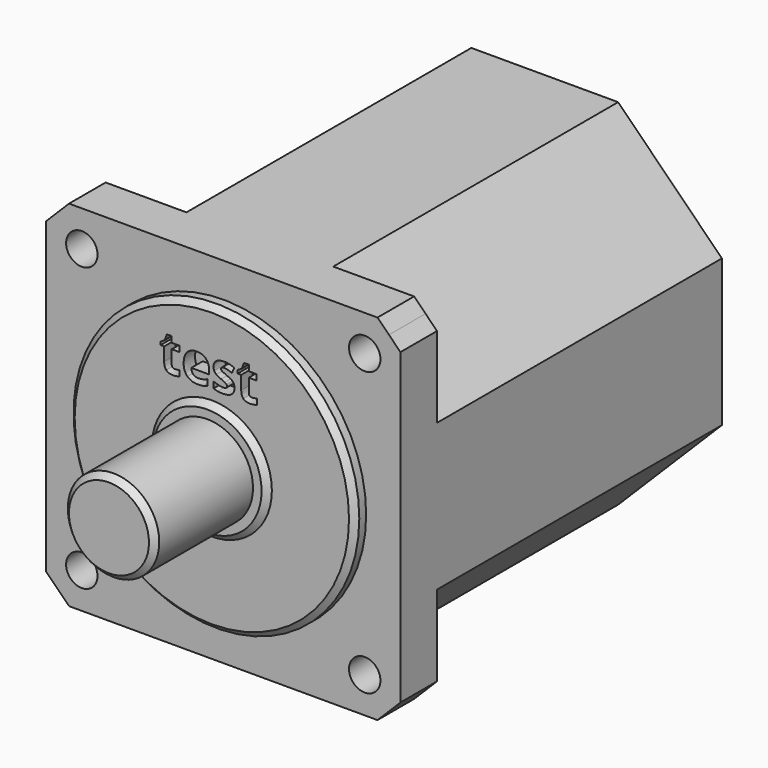
from build123d import *

# Parameters (mm, degrees)
F1_DEPTH  = 70.3
F2_DEPTH  = 62.3
F3_DEPTH  = 62.3
F4_R      = 2.75
F5_DEPTH  = 8
F4_R_2    = 25
F4_R_3    = 8
F6_DEPTH  = 2.5
F7_DEPTH  = 70.301
F8_R      = 10.5
F8_R_2    = 8
F9_DEPTH  = 1
F10_SIZE  = 0.99999
F11_SIZE  = 1
F12_DEPTH = 25
F13_SIZE  = 1


# Not quite as in the source:
# - a fillet or chamfer is up to 0.001 mm smaller than in the source, because OpenCascade refuses the exact size


with BuildPart() as f1:
    # F0 (on Front) → F1 (new body)
    with BuildSketch(Plane.XZ):
        Polygon((12.841, -31), (31, -31), (31, -12.841), align=None)
        Polygon((-12.841, -31), (12.841, -31), (31, -12.841), (31, 12.841), (12.841, 31), (-12.841, 31), (-31, 12.841), (-31, -12.841), align=None)
        Polygon((-31, -31), (-12.841, -31), (-31, -12.841), align=None)
        Polygon((12.841, 31), (31, 12.841), (31, 31), align=None)
        Polygon((-31, 31), (-31, 12.841), (-12.841, 31), align=None)
    extrude(amount=F1_DEPTH)

    # F0 (on Front) → F2 (cut)
    with BuildSketch(Plane.XZ):
        Polygon((12.841, 31), (31, 12.841), (31, 31), align=None)
    extrude(amount=F2_DEPTH, mode=Mode.SUBTRACT)

    # F0 (on Front) → F3 (cut)
    with BuildSketch(Plane.XZ):
        Polygon((-31, 31), (-31, 12.841), (-12.841, 31), align=None)
        Polygon((-31, -31), (-12.841, -31), (-31, -12.841), align=None)
        Polygon((12.841, -31), (31, -31), (31, -12.841), align=None)
    extrude(amount=F3_DEPTH, mode=Mode.SUBTRACT)

    # F4 (on face) → F5 (cut)
    with BuildSketch(Plane.XZ.offset(70.3)):
        with Locations((-24.7487373415, 24.7487373415)):
            Circle(F4_R)
        with Locations((24.7487373415, 24.7487373415)):
            Circle(F4_R)
        with Locations((24.7487373415, -24.7487373415)):
            Circle(F4_R)
        with Locations((-24.7487373415, -24.7487373415)):
            Circle(F4_R)
    extrude(amount=-F5_DEPTH, mode=Mode.SUBTRACT)

    # F4 (on face) → F6 (join)
    with BuildSketch(Plane.XZ.offset(70.3)):
        Circle(F4_R_2)
        with BuildLine():
            add(Edge.make_bspline(
                [(-6.8632484674, 13.3325467897), (-6.7054646432, 13.1982921323), (-6.4452597403, 13.1982921323)],
                knots=[0, 0, 0, 1, 1, 1], degree=2))
            add(Edge.make_bspline(
                [(-6.4452597403, 13.1982921323), (-6.099242582, 13.1982921323), (-5.6148185605, 13.3491556133)],
                knots=[0, 0, 0, 1, 1, 1], degree=2))
            Line((-5.6148185605, 13.3491556133), (-5.6148185605, 12.3678509525))
            add(Edge.make_bspline(
                [(-5.6148185605, 12.3678509525), (-6.1075469938, 12.1463999712), (-6.8258786143, 12.1463999712)],
                knots=[0, 0, 0, 1, 1, 1], degree=2))
            add(Edge.make_bspline(
                [(-6.8258786143, 12.1463999712), (-7.6175658724, 12.1463999712), (-7.9788077855, 12.5470878405)],
                knots=[0, 0, 0, 1, 1, 1], degree=2))
            add(Edge.make_bspline(
                [(-7.9788077855, 12.5470878405), (-8.3400496987, 12.9477757097), (-8.3400496987, 13.7477673796)],
                knots=[0, 0, 0, 1, 1, 1], degree=2))
            Line((-8.3400496987, 13.7477673796), (-8.3400496987, 16.0785389574))
            Line((-8.3400496987, 16.0785389574), (-8.9711849954, 16.0785389574))
            Line((-8.9711849954, 16.0785389574), (-8.9711849954, 16.6363186165))
            Line((-8.9711849954, 16.6363186165), (-8.2445489631, 17.0778365104))
            Line((-8.2445489631, 17.0778365104), (-7.863930089, 18.0992791615))
            Line((-7.863930089, 18.0992791615), (-7.0210322916, 18.0992791615))
            Line((-7.0210322916, 18.0992791615), (-7.0210322916, 17.0695320986))
            Line((-7.0210322916, 17.0695320986), (-5.6674131685, 17.0695320986))
            Line((-5.6674131685, 17.0695320986), (-5.6674131685, 16.0785389574))
            Line((-5.6674131685, 16.0785389574), (-7.0210322916, 16.0785389574))
            Line((-7.0210322916, 16.0785389574), (-7.0210322916, 13.7477673796))
            add(Edge.make_bspline(
                [(-7.0210322916, 13.7477673796), (-7.0210322916, 13.4668014471), (-6.8632484674, 13.3325467897)],
                knots=[0, 0, 0, 1, 1, 1], degree=2))
        make_face(mode=Mode.SUBTRACT)
        with BuildLine():
            add(Edge.make_bspline(
                [(-1.4889099657, 12.2308281579), (-1.8819854575, 12.1463999712), (-2.449453597, 12.1463999712)],
                knots=[0, 0, 0, 1, 1, 1], degree=2))
            add(Edge.make_bspline(
                [(-2.449453597, 12.1463999712), (-3.6162234545, 12.1463999712), (-4.2736560552, 12.7913759542)],
                knots=[0, 0, 0, 1, 1, 1], degree=2))
            add(Edge.make_bspline(
                [(-4.2736560552, 12.7913759542), (-4.9310886558, 13.4363519371), (-4.9310886558, 14.616962481)],
                knots=[0, 0, 0, 1, 1, 1], degree=2))
            add(Edge.make_bspline(
                [(-4.9310886558, 14.616962481), (-4.9310886558, 15.8321747408), (-4.323482526, 16.4958356503)],
                knots=[0, 0, 0, 1, 1, 1], degree=2))
            add(Edge.make_bspline(
                [(-4.323482526, 16.4958356503), (-3.7158763961, 17.1594965597), (-2.6432232056, 17.1594965597)],
                knots=[0, 0, 0, 1, 1, 1], degree=2))
            add(Edge.make_bspline(
                [(-2.6432232056, 17.1594965597), (-1.6190124172, 17.1594965597), (-1.0480841061, 16.576111631)],
                knots=[0, 0, 0, 1, 1, 1], degree=2))
            add(Edge.make_bspline(
                [(-1.0480841061, 16.576111631), (-0.477155795, 15.9927267022), (-0.477155795, 14.9629796393)],
                knots=[0, 0, 0, 1, 1, 1], degree=2))
            Line((-0.477155795, 14.9629796393), (-0.477155795, 14.3221558622))
            Line((-0.477155795, 14.3221558622), (-3.595462425, 14.3221558622))
            add(Edge.make_bspline(
                [(-3.595462425, 14.3221558622), (-3.5733173269, 13.7602239972), (-3.2619018845, 13.4446563489)],
                knots=[0, 0, 0, 1, 1, 1], degree=2))
            add(Edge.make_bspline(
                [(-3.2619018845, 13.4446563489), (-2.9504864421, 13.1290887006), (-2.3885545771, 13.1290887006)],
                knots=[0, 0, 0, 1, 1, 1], degree=2))
            add(Edge.make_bspline(
                [(-2.3885545771, 13.1290887006), (-1.9511888891, 13.1290887006), (-1.5622656032, 13.2197451961)],
                knots=[0, 0, 0, 1, 1, 1], degree=2))
            add(Edge.make_bspline(
                [(-1.5622656032, 13.2197451961), (-1.1733423174, 13.3104016915), (-0.7498173157, 13.5097075747)],
                knots=[0, 0, 0, 1, 1, 1], degree=2))
            Line((-0.7498173157, 13.5097075747), (-0.7498173157, 12.4882649236))
            add(Edge.make_bspline(
                [(-0.7498173157, 12.4882649236), (-1.0958344739, 12.3152563445), (-1.4889099657, 12.2308281579)],
                knots=[0, 0, 0, 1, 1, 1], degree=2))
        make_face(mode=Mode.SUBTRACT)
        Circle(F4_R_3, mode=Mode.SUBTRACT)
        with BuildLine():
            add(Edge.make_bspline(
                [(3.843906477, 14.2882461807), (3.9698567226, 14.028733312), (3.9698567226, 13.6702595361)],
                knots=[0, 0, 0, 1, 1, 1], degree=2))
            add(Edge.make_bspline(
                [(3.9698567226, 13.6702595361), (3.9698567226, 12.9256306116), (3.4529070882, 12.5360152914)],
                knots=[0, 0, 0, 1, 1, 1], degree=2))
            add(Edge.make_bspline(
                [(3.4529070882, 12.5360152914), (2.9359574538, 12.1463999712), (1.9062103909, 12.1463999712)],
                knots=[0, 0, 0, 1, 1, 1], degree=2))
            add(Edge.make_bspline(
                [(1.9062103909, 12.1463999712), (1.3788802417, 12.1463999712), (1.0065657795, 12.2183715402)],
                knots=[0, 0, 0, 1, 1, 1], degree=2))
            add(Edge.make_bspline(
                [(1.0065657795, 12.2183715402), (0.6342513172, 12.2903431091), (0.3103792571, 12.4287499724)],
                knots=[0, 0, 0, 1, 1, 1], degree=2))
            Line((0.3103792571, 12.4287499724), (0.3103792571, 13.5180119865))
            add(Edge.make_bspline(
                [(0.3103792571, 13.5180119865), (0.6771574448, 13.3450034074), (1.1380522996, 13.2280496079)],
                knots=[0, 0, 0, 1, 1, 1], degree=2))
            add(Edge.make_bspline(
                [(1.1380522996, 13.2280496079), (1.5989471544, 13.1110958084), (1.9491165185, 13.1110958084)],
                knots=[0, 0, 0, 1, 1, 1], degree=2))
            add(Edge.make_bspline(
                [(1.9491165185, 13.1110958084), (2.667448139, 13.1110958084), (2.667448139, 13.5263163983)],
                knots=[0, 0, 0, 1, 1, 1], degree=2))
            add(Edge.make_bspline(
                [(2.667448139, 13.5263163983), (2.667448139, 13.6827161538), (2.5719474033, 13.7802929924)],
                knots=[0, 0, 0, 1, 1, 1], degree=2))
            add(Edge.make_bspline(
                [(2.5719474033, 13.7802929924), (2.4764466677, 13.877869831), (2.243231103, 14.0010519394)],
                knots=[0, 0, 0, 1, 1, 1], degree=2))
            add(Edge.make_bspline(
                [(2.243231103, 14.0010519394), (2.0100155384, 14.1242340477), (1.6210922525, 14.2875541464)],
                knots=[0, 0, 0, 1, 1, 1], degree=2))
            add(Edge.make_bspline(
                [(1.6210922525, 14.2875541464), (1.0633125934, 14.5214617454), (0.8010315875, 14.7207676285)],
                knots=[0, 0, 0, 1, 1, 1], degree=2))
            add(Edge.make_bspline(
                [(0.8010315875, 14.7207676285), (0.5387505816, 14.9200735117), (0.4204127134, 15.1775102774)],
                knots=[0, 0, 0, 1, 1, 1], degree=2))
            add(Edge.make_bspline(
                [(0.4204127134, 15.1775102774), (0.3020748453, 15.4349470431), (0.3020748453, 15.8100296426)],
                knots=[0, 0, 0, 1, 1, 1], degree=2))
            add(Edge.make_bspline(
                [(0.3020748453, 15.8100296426), (0.3020748453, 16.4550056256), (0.8010315875, 16.8072510927)],
                knots=[0, 0, 0, 1, 1, 1], degree=2))
            add(Edge.make_bspline(
                [(0.8010315875, 16.8072510927), (1.2999883297, 17.1594965597), (2.2176258333, 17.1594965597)],
                knots=[0, 0, 0, 1, 1, 1], degree=2))
            add(Edge.make_bspline(
                [(2.2176258333, 17.1594965597), (3.0909731407, 17.1594965597), (3.9172621146, 16.7788776857)],
                knots=[0, 0, 0, 1, 1, 1], degree=2))
            Line((3.9172621146, 16.7788776857), (3.5200344169, 15.8280225349))
            add(Edge.make_bspline(
                [(3.5200344169, 15.8280225349), (3.1560243664, 15.9830382217), (2.8404567181, 16.0826911633)],
                knots=[0, 0, 0, 1, 1, 1], degree=2))
            add(Edge.make_bspline(
                [(2.8404567181, 16.0826911633), (2.5248890698, 16.1823441049), (2.1954807352, 16.1823441049)],
                knots=[0, 0, 0, 1, 1, 1], degree=2))
            add(Edge.make_bspline(
                [(2.1954807352, 16.1823441049), (1.6114037721, 16.1823441049), (1.6114037721, 15.8667764566)],
                knots=[0, 0, 0, 1, 1, 1], degree=2))
            add(Edge.make_bspline(
                [(1.6114037721, 15.8667764566), (1.6114037721, 15.6896156716), (1.7996371062, 15.5595132201)],
                knots=[0, 0, 0, 1, 1, 1], degree=2))
            add(Edge.make_bspline(
                [(1.7996371062, 15.5595132201), (1.9878704402, 15.4294107686), (2.6245420114, 15.1747421401)],
                knots=[0, 0, 0, 1, 1, 1], degree=2))
            add(Edge.make_bspline(
                [(2.6245420114, 15.1747421401), (3.1906260823, 14.944986747), (3.4542911568, 14.7463728982)],
                knots=[0, 0, 0, 1, 1, 1], degree=2))
            add(Edge.make_bspline(
                [(3.4542911568, 14.7463728982), (3.7179562314, 14.5477590494), (3.843906477, 14.2882461807)],
                knots=[0, 0, 0, 1, 1, 1], degree=2))
        make_face(mode=Mode.SUBTRACT)
        with BuildLine():
            add(Edge.make_bspline(
                [(6.6175800174, 13.3325467897), (6.7753638416, 13.1982921323), (7.0355687446, 13.1982921323)],
                knots=[0, 0, 0, 1, 1, 1], degree=2))
            add(Edge.make_bspline(
                [(7.0355687446, 13.1982921323), (7.3815859028, 13.1982921323), (7.8660099243, 13.3491556133)],
                knots=[0, 0, 0, 1, 1, 1], degree=2))
            Line((7.8660099243, 13.3491556133), (7.8660099243, 12.3678509525))
            add(Edge.make_bspline(
                [(7.8660099243, 12.3678509525), (7.373281491, 12.1463999712), (6.6549498705, 12.1463999712)],
                knots=[0, 0, 0, 1, 1, 1], degree=2))
            add(Edge.make_bspline(
                [(6.6549498705, 12.1463999712), (5.8632626125, 12.1463999712), (5.5020206993, 12.5470878405)],
                knots=[0, 0, 0, 1, 1, 1], degree=2))
            add(Edge.make_bspline(
                [(5.5020206993, 12.5470878405), (5.1407787861, 12.9477757097), (5.1407787861, 13.7477673796)],
                knots=[0, 0, 0, 1, 1, 1], degree=2))
            Line((5.1407787861, 13.7477673796), (5.1407787861, 16.0785389574))
            Line((5.1407787861, 16.0785389574), (4.5096434895, 16.0785389574))
            Line((4.5096434895, 16.0785389574), (4.5096434895, 16.6363186165))
            Line((4.5096434895, 16.6363186165), (5.2362795217, 17.0778365104))
            Line((5.2362795217, 17.0778365104), (5.6168983958, 18.0992791615))
            Line((5.6168983958, 18.0992791615), (6.4597961933, 18.0992791615))
            Line((6.4597961933, 18.0992791615), (6.4597961933, 17.0695320986))
            Line((6.4597961933, 17.0695320986), (7.8134153163, 17.0695320986))
            Line((7.8134153163, 17.0695320986), (7.8134153163, 16.0785389574))
            Line((7.8134153163, 16.0785389574), (6.4597961933, 16.0785389574))
            Line((6.4597961933, 16.0785389574), (6.4597961933, 13.7477673796))
            add(Edge.make_bspline(
                [(6.4597961933, 13.7477673796), (6.4597961933, 13.4668014471), (6.6175800174, 13.3325467897)],
                knots=[0, 0, 0, 1, 1, 1], degree=2))
        make_face(mode=Mode.SUBTRACT)
    extrude(amount=F6_DEPTH)

    # F4 (on face) → F7 (cut, through all)
    with BuildSketch(Plane.XZ.offset(70.3)):
        Polygon((26.9827560573, 31), (28.9913780286, 28.9913780286), (31, 26.9827560573), (31, 31), align=None)
        Polygon((31, -31), (31, -26.9827560573), (28.9913780286, -28.9913780286), (26.9827560573, -31), align=None)
        Polygon((-31, -31), (-26.9827560573, -31), (-28.9913780286, -28.9913780286), (-31, -26.9827560573), align=None)
        Polygon((-28.9913780286, 28.9913780286), (-26.9827560573, 31), (-31, 31), (-31, 26.9827560573), align=None)
    extrude(amount=-F7_DEPTH, mode=Mode.SUBTRACT)

    # F8 (on face) → F9 (join)
    with BuildSketch(Plane.XZ.offset(72.8)):
        Circle(F8_R)
        Circle(F8_R_2, mode=Mode.SUBTRACT)
    extrude(amount=F9_DEPTH)

    # F10 (size 1 in the source; OpenCascade refuses exactly that, so slightly less here)
    f10_edges = [f1.edges().sort_by_distance(p)[0] for p in [
        (-10.5, -73.8, 0),
    ]]
    chamfer(f10_edges, length=F10_SIZE)

    # F11
    f11_edges = [f1.edges().sort_by_distance(p)[0] for p in [
        (-25, -72.8, 0),
    ]]
    chamfer(f11_edges, length=F11_SIZE)

    # F4 (on face) → F12 (join)
    with BuildSketch(Plane.XZ.offset(70.3)):
        Circle(F4_R_3)
    extrude(amount=F12_DEPTH)

    # F13
    f13_edges = [f1.edges().sort_by_distance(p)[0] for p in [
        (-8, -95.3, 0),
    ]]
    chamfer(f13_edges, length=F13_SIZE)


solid = f1.part
